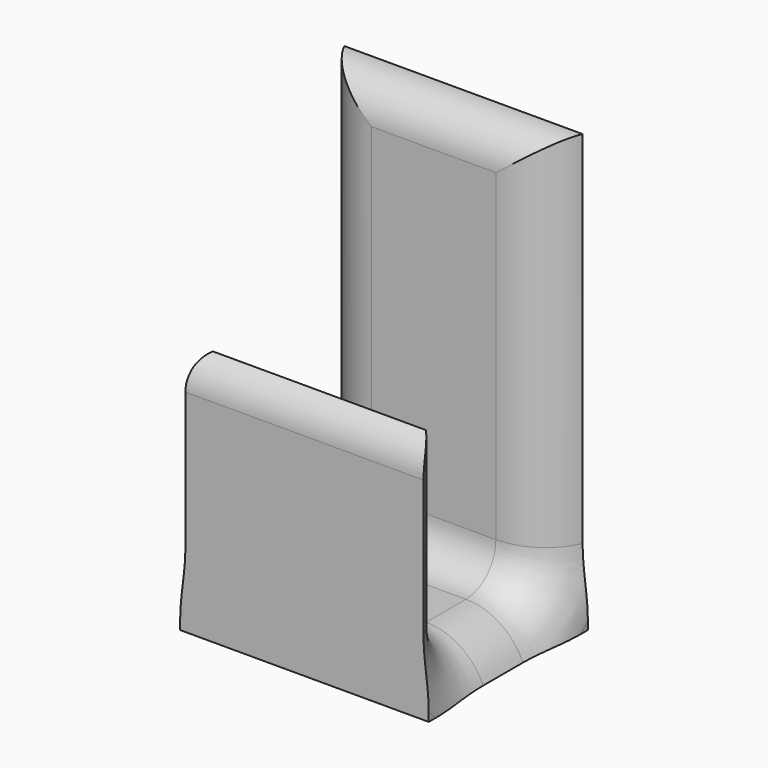
from build123d import *

# Parameters (mm, degrees)
F1_DEPTH     = 20
F2_T1_DEPTH  = 20
F2_T3_DEPTH  = 35
F3_T1_DEPTH  = 4
F3_T3_DEPTH  = 23.5
F3_T5_DEPTH  = 38.5
F3_T8_ANGLE  = 89.9999999987
F3_T10_ANGLE = 89.9999999987
F3_T12_ANGLE = 89.9999999987
F3_T14_ANGLE = 89.9999999987
F3_T18_ANGLE = 359.64
F3_S19_R     = 5
F3_T20_DEPTH = 6
F3_T24_ANGLE = 359.64
F3_S25_R     = 5
F3_T26_DEPTH = 6
F3_T30_ANGLE = 328.8283154119
F3_S31_R     = 5
F3_T32_DEPTH = 6
F3_T36_ANGLE = 328.8283154119
F3_S37_R     = 5
F3_T38_DEPTH = 6


# Not quite as in the source:
# - a fillet or chamfer that OpenCascade refuses, or shapes differently, is made with other operations: its cross-section is extruded or revolved along the edge and cut away or added


with BuildPart() as f1:
    # F0 (on Right) → F1 (new body)
    with BuildSketch(Plane.YZ):
        Polygon((0, -10.05617938), (0, 24.94382062), (-3, 24.94382062), (-3, -7.05617938), (-13, -7.05617938), (-13, 9.94382062), (-16, 9.94382062), (-16, -10.05617938), align=None)
    extrude(amount=F1_DEPTH)

    # F2: fillet of radius 3 on 5 edges, made by hand

    # F2_s2 → F2_t1 (join)
    with BuildSketch(Plane.YZ):
        with BuildLine():
            ThreePointArc((-10, -7.05617938), (-12.1213203436, -6.1774997235), (-13, -4.05617938))
            Line((-13, -4.05617938), (-13, -7.05617938))
            Line((-13, -7.05617938), (-10, -7.05617938))
        make_face()
        with BuildLine():
            ThreePointArc((-3, -4.05617938), (-3.8786796564, -6.1774997235), (-6, -7.05617938))
            Line((-6, -7.05617938), (-3, -7.05617938))
            Line((-3, -7.05617938), (-3, -4.05617938))
        make_face()
    extrude(amount=F2_T1_DEPTH)

    # F2_s4 → F2_t3 (cut)
    with BuildSketch(Plane.YZ.offset(-7.5)):
        with BuildLine():
            ThreePointArc((0, 24.94382062), (-2.1213203436, 24.0651409636), (-3, 21.94382062))
            Line((-3, 21.94382062), (-3, 24.94382062))
            Line((-3, 24.94382062), (0, 24.94382062))
        make_face()
        with BuildLine():
            ThreePointArc((-13, 6.94382062), (-13.8786796564, 9.0651409636), (-16, 9.94382062))
            Line((-16, 9.94382062), (-13, 9.94382062))
            Line((-13, 9.94382062), (-13, 6.94382062))
        make_face()
        with BuildLine():
            ThreePointArc((-16, 6.94382062), (-15.1213203436, 9.0651409636), (-13, 9.94382062))
            Line((-13, 9.94382062), (-16, 9.94382062))
            Line((-16, 9.94382062), (-16, 6.94382062))
        make_face()
    extrude(amount=F2_T3_DEPTH, mode=Mode.SUBTRACT)

    # F3: fillet of radius 5 on 4 edges, made by hand

    # F3_s2 → F3_t1 (cut)
    with BuildSketch(Plane.XZ.offset(6)):
        with BuildLine():
            ThreePointArc((20, -12.05617938), (18.5355339059, -8.520645474), (15, -7.05617938))
            Line((15, -7.05617938), (20, -7.05617938))
            Line((20, -7.05617938), (20, -12.05617938))
        make_face()
        with BuildLine():
            ThreePointArc((0, -12.05617938), (1.4644660941, -8.520645474), (5, -7.05617938))
            Line((5, -7.05617938), (0, -7.05617938))
            Line((0, -7.05617938), (0, -12.05617938))
        make_face()
    extrude(amount=F3_T1_DEPTH, mode=Mode.SUBTRACT)

    # F3_s4 → F3_t3 (cut)
    with BuildSketch(Plane.XY.offset(-4.05617938)):
        with BuildLine():
            ThreePointArc((20, -18), (18.5355339059, -14.4644660941), (15, -13))
            Line((15, -13), (20, -13))
            Line((20, -13), (20, -18))
        make_face()
        with BuildLine():
            ThreePointArc((0, -18), (1.4644660941, -14.4644660941), (5, -13))
            Line((5, -13), (0, -13))
            Line((0, -13), (0, -18))
        make_face()
    extrude(amount=F3_T3_DEPTH, mode=Mode.SUBTRACT)

    # F3_s6 → F3_t5 (cut)
    with BuildSketch(Plane.XY.offset(-4.05617938)):
        with BuildLine():
            ThreePointArc((20, 2), (18.5355339059, -1.5355339059), (15, -3))
            Line((15, -3), (20, -3))
            Line((20, -3), (20, 2))
        make_face()
        with BuildLine():
            ThreePointArc((0, 2), (1.4644660941, -1.5355339059), (5, -3))
            Line((5, -3), (0, -3))
            Line((0, -3), (0, 2))
        make_face()
    extrude(amount=F3_T5_DEPTH, mode=Mode.SUBTRACT)

    # F3_s7 → F3_t8 (revolve, cut)
    with BuildSketch(Plane.XY.offset(-4.05617938)):
        with BuildLine():
            ThreePointArc((0, 2), (1.4644660941, -1.5355339059), (5, -3))
            Line((5, -3), (0, -3))
            Line((0, -3), (0, 2))
        make_face()
    revolve(axis=Axis((0, -6, -4.05617938), (-1, 0, 0)), revolution_arc=F3_T8_ANGLE, mode=Mode.SUBTRACT)

    # F3_s9 → F3_t10 (revolve, cut)
    with BuildSketch(Plane.XY.offset(-4.05617938)):
        with BuildLine():
            ThreePointArc((20, 2), (18.5355339059, -1.5355339059), (15, -3))
            Line((15, -3), (20, -3))
            Line((20, -3), (20, 2))
        make_face()
    revolve(axis=Axis((20, -6, -4.05617938), (-1, 0, 0)), revolution_arc=F3_T10_ANGLE, mode=Mode.SUBTRACT)

    # F3_s11 → F3_t12 (revolve, cut)
    with BuildSketch(Plane.XZ.offset(10)):
        with BuildLine():
            ThreePointArc((0, -12.05617938), (1.4644660941, -8.5206454741), (5, -7.05617938))
            Line((5, -7.05617938), (0, -7.05617938))
            Line((0, -7.05617938), (0, -12.05617938))
        make_face()
    revolve(axis=Axis((0, -10, -4.05617938), (-1, 0, 0)), revolution_arc=F3_T12_ANGLE, mode=Mode.SUBTRACT)

    # F3_s13 → F3_t14 (revolve, cut)
    with BuildSketch(Plane.XZ.offset(10)):
        with BuildLine():
            ThreePointArc((20, -12.05617938), (18.5355339059, -8.5206454741), (15, -7.05617938))
            Line((15, -7.05617938), (20, -7.05617938))
            Line((20, -7.05617938), (20, -12.05617938))
        make_face()
    revolve(axis=Axis((20, -10, -4.05617938), (-1, 0, 0)), revolution_arc=F3_T14_ANGLE, mode=Mode.SUBTRACT)


with BuildPart() as f3_tool16:
    # F3_s17 → F3_t18 (revolve)
    with BuildSketch(Plane(origin=(0, 0.0429965174, 6.8430181729), x_dir=(1, 0, 0), z_dir=(0, 0.006283144, 0.9999802609))):
        with BuildLine():
            ThreePointArc((19.5825756949, -16.0433131985), (17.7386127875, -13.8600130659), (15, -13.0433131986))
            Line((15, -13.0433131986), (20, -13.0433131986))
            Line((20, -13.0433131986), (20, -16.0433131985))
            Line((20, -16.0433131985), (19.5825756949, -16.0433131985))
        make_face()
    revolve(axis=Axis((20, -15.9999999999, 6.9438206201), (-1, 0, 0)), revolution_arc=F3_T18_ANGLE)

    # F3_s19 → F3_t20 (cut, symmetric)
    with BuildSketch(Plane.XY.offset(6.9)):
        with Locations((15, -18)):
            Circle(F3_S19_R)
    extrude(amount=F3_T20_DEPTH, both=True, mode=Mode.SUBTRACT)


with BuildPart() as f1_1:
    add(f1.part)

    # F3_t15: cut F3_tool16
    add(f3_tool16.part, mode=Mode.SUBTRACT)


with BuildPart() as f3_tool22:
    # F3_s23 → F3_t24 (revolve)
    with BuildSketch(Plane(origin=(0, 0.0429965174, 6.8430181729), x_dir=(1, 0, 0), z_dir=(0, 0.006283144, 0.9999802609))):
        with BuildLine():
            ThreePointArc((0.4174243051, -16.0433131985), (2.2613872125, -13.8600130659), (5, -13.0433131986))
            Line((5, -13.0433131986), (0, -13.0433131986))
            Line((0, -13.0433131986), (0, -16.0433131985))
            Line((0, -16.0433131985), (0.4174243051, -16.0433131985))
        make_face()
    revolve(axis=Axis((0, -15.9999999999, 6.9438206201), (-1, 0, 0)), revolution_arc=F3_T24_ANGLE)

    # F3_s25 → F3_t26 (cut, symmetric)
    with BuildSketch(Plane.XY.offset(6.9)):
        with Locations((5, -18)):
            Circle(F3_S25_R)
    extrude(amount=F3_T26_DEPTH, both=True, mode=Mode.SUBTRACT)


with BuildPart() as f1_2:
    add(f1_1.part)

    # F3_t21: cut F3_tool22
    add(f3_tool22.part, mode=Mode.SUBTRACT)


with BuildPart() as f3_tool28:
    # F3_s29 → F3_t30 (revolve)
    with BuildSketch(Plane.XY.offset(21.9438206201)):
        with BuildLine():
            ThreePointArc((15, -3), (17.7386127875, -2.1833001327), (19.5825756949, -1e-10))
            Line((19.5825756949, -1e-10), (20, -1e-10))
            Line((20, -1e-10), (20, -3))
            Line((20, -3), (15, -3))
        make_face()
    revolve(axis=Axis((20, -1e-10, 21.9438206201), (-1, 0, 0)), revolution_arc=F3_T30_ANGLE)

    # F3_s31 → F3_t32 (cut, symmetric)
    with BuildSketch(Plane.XY.offset(21.9)):
        with Locations((15, 2)):
            Circle(F3_S31_R)
    extrude(amount=F3_T32_DEPTH, both=True, mode=Mode.SUBTRACT)


with BuildPart() as f1_3:
    add(f1_2.part)

    # F3_t27: cut F3_tool28
    add(f3_tool28.part, mode=Mode.SUBTRACT)


with BuildPart() as f3_tool34:
    # F3_s35 → F3_t36 (revolve)
    with BuildSketch(Plane.XY.offset(21.9438206201)):
        with BuildLine():
            ThreePointArc((5, -3), (2.2613872125, -2.1833001327), (0.4174243051, -1e-10))
            Line((0.4174243051, -1e-10), (0, -1e-10))
            Line((0, -1e-10), (0, -3))
            Line((0, -3), (5, -3))
        make_face()
    revolve(axis=Axis((0, -1e-10, 21.9438206201), (-1, 0, 0)), revolution_arc=F3_T36_ANGLE)

    # F3_s37 → F3_t38 (cut, symmetric)
    with BuildSketch(Plane.XY.offset(21.9)):
        with Locations((5, 2)):
            Circle(F3_S37_R)
    extrude(amount=F3_T38_DEPTH, both=True, mode=Mode.SUBTRACT)


with BuildPart() as f1_4:
    add(f1_3.part)

    # F3_t33: cut F3_tool34
    add(f3_tool34.part, mode=Mode.SUBTRACT)


solid = f1_4.part
